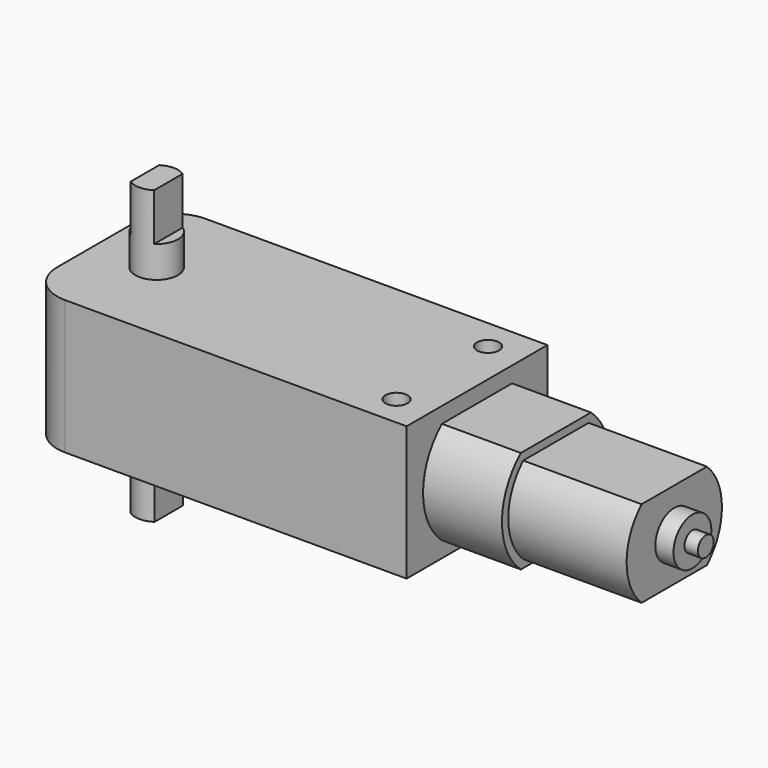
from build123d import *

# Parameters (mm, degrees)
F0_W         = 7.9850807097
F0_H         = 22.3
F0_R         = 1.4
F0_R_2       = 2.7
F1_DEPTH     = 8.5
F0_W_2       = 1.8826620857
F0_H_2       = 1.8826614193
F2_DEPTH     = 1.5
F3_DEPTH     = 18.5
F5_DEPTH     = 10
F6_T         = 1
F6_T3_DEPTH  = 13.109005356
F6_T5_DEPTH  = 5
F6_T7_DEPTH  = 3.8826614193
F6_T10_ANGLE = 98.969647871
F6_T12_ANGLE = 98.969647871
F8_DEPTH     = 15
F9_R         = 3
F9_R_2       = 1.25
F10_DEPTH    = 2.3
F11_DEPTH    = 4
F13_DEPTH    = 6
F15_DEPTH    = 6


# Not quite as in the source:
# - a shell that OpenCascade refuses in one call is made with other operations: the cavity is built on its own and cut out


with BuildPart() as f1:
    # F0 (on Top) → F1 (new body, symmetric)
    with BuildSketch(Plane.XY):
        with Locations((20.1574596452, 0)):
            Rectangle(F0_W, F0_H)
        with Locations((19.75, -7.25)):
            Circle(F0_R, mode=Mode.SUBTRACT)
        with Locations((19.75, 7.25)):
            Circle(F0_R, mode=Mode.SUBTRACT)
        with BuildLine():
            Line((-19.15, -11.15), (16.1649192903, -11.15))
            Line((16.1649192903, -11.15), (16.1649192903, 11.15))
            Line((16.1649192903, 11.15), (-19.15, 11.15))
            ThreePointArc((-19.15, 11.15), (-22.6855339059, 9.6855339059), (-24.15, 6.15))
            Line((-24.15, 6.15), (-24.15, 1.8826614193))
            Line((-24.15, 1.8826614193), (-24.15, 0))
            Line((-24.15, 0), (-24.15, -6.15))
            ThreePointArc((-24.15, -6.15), (-22.6855339059, -9.6855339059), (-19.15, -11.15))
        make_face()
        with Locations((-16.45, 0)):
            Circle(F0_R_2, mode=Mode.SUBTRACT)
    extrude(amount=F1_DEPTH, both=True)

    # F0 (on Top) → F2 (join, symmetric)
    with BuildSketch(Plane.XY):
        with Locations((-25.0913310429, 0.9413307097)):
            Rectangle(F0_W_2, F0_H_2)
    extrude(amount=F2_DEPTH, both=True)

    # F4 (on face) → F5 (join)
    with BuildSketch(Plane.YZ.offset(24.15)):
        with BuildLine():
            Line((5.554502678, 6.5), (-5.554502678, 6.5))
            ThreePointArc((-5.554502678, 6.5), (-8.55, 0), (-5.554502678, -6.5))
            Line((-5.554502678, -6.5), (5.554502678, -6.5))
            ThreePointArc((5.554502678, -6.5), (8.55, 0), (5.554502678, 6.5))
        make_face()
    extrude(amount=F5_DEPTH)

    # F6: shell of thickness 1, made by hand


with BuildPart() as f3:
    # F0 (on Top) → F3 (new body, symmetric)
    with BuildSketch(Plane.XY):
        with Locations((-16.45, 0)):
            Circle(F0_R_2)
    extrude(amount=F3_DEPTH, both=True)

    # F12 (on face) → F13 (cut)
    with BuildSketch(Plane.XY.offset(18.5)):
        with BuildLine():
            ThreePointArc((-17.9390255067, 2.2522884008), (-19.15, 0), (-17.9390255067, -2.2522884008))
            Line((-17.9390255067, -2.2522884008), (-17.9390255067, 2.2522884008))
        make_face()
        with BuildLine():
            Line((-14.9609744933, 2.2522884008), (-14.9609744933, -2.2522884008))
            ThreePointArc((-14.9609744933, -2.2522884008), (-14.0719368314, -1.2785990638), (-13.75, 0))
            ThreePointArc((-13.75, 0), (-14.0719368314, 1.2785990638), (-14.9609744933, 2.2522884008))
        make_face()
    extrude(amount=-F13_DEPTH, mode=Mode.SUBTRACT)

    # F14 (on face) → F15 (cut)
    with BuildSketch(Plane(origin=(0, 0, -18.5), x_dir=(1, 0, 0), z_dir=(0, 0, -1))):
        with BuildLine():
            Line((-17.9761945408, -2.2272696792), (-17.9761945408, 2.2272696792))
            ThreePointArc((-17.9761945408, 2.2272696792), (-19.15, 0), (-17.9761945408, -2.2272696792))
        make_face()
        with BuildLine():
            ThreePointArc((-13.75, 0), (-14.0614099075, 1.2588238042), (-14.9238054592, 2.2272696792))
            Line((-14.9238054592, 2.2272696792), (-14.9238054592, -2.2272696792))
            ThreePointArc((-14.9238054592, -2.2272696792), (-14.0614099075, -1.2588238042), (-13.75, 0))
        make_face()
    extrude(amount=-F15_DEPTH, mode=Mode.SUBTRACT)


with BuildPart() as f6_core1:
    # F6_t2: copy of F1
    add(f1.part)

    # the walls: a layer under each face that stays
    f6_faces = [f6_core1.faces().sort_by_distance(p)[0] for p in [
        (24.15, -7.4333333333, -5.6666666667),
        (0, 0, -8.5),
        (2.5, -11.15, 0),
        (2.5, 11.15, 0),
        (0, 0, 8.5),
        (29.15, 0, -6.5),
        (29.15, 8.55, 0),
        (29.15, 0, 6.5),
        (29.15, -8.55, 0),
        (-22.6855339059, 9.6855339059, 0),
        (-24.15, 4.1, -5.6666666667),
        (-22.6855339059, -9.6855339059, 0),
        (18.35, -7.25, 0),
        (18.35, 7.25, 0),
        (-19.15, 0, 0),
        (-25.0913310429, 1.8826614193, 0),
        (-25.0913310429, 0.9413307097, -1.5),
        (-25.0913310429, 0, 0),
        (-25.0913310429, 0.9413307097, 1.5),
        (-26.0326620857, 0.9413307097, 0),
    ]]
    thicken(f6_faces, amount=-F6_T, mode=Mode.SUBTRACT)

    # F6_s4 → F6_t3 (cut)
    with BuildSketch(Plane.XZ.offset(-6.554502678)):
        Polygon((24.16, -6.51), (23.15, -6.5), (23.15, -5.5), (24.15, -5.5), align=None)
        Polygon((24.16, 6.51), (23.15, 6.5), (23.15, 5.5), (24.15, 5.5), align=None)
    extrude(amount=F6_T3_DEPTH, mode=Mode.SUBTRACT)

    # F6_s6 → F6_t5 (cut)
    with BuildSketch(Plane.XY.offset(-2.5)):
        Polygon((-24.16, 1.8926614193), (-23.15, 1.8826614193), (-23.15, 0.8826614193), (-24.15, 0.8826614193), align=None)
        Polygon((-24.16, -0.01), (-23.15, 0), (-23.15, 1), (-24.15, 1), align=None)
    extrude(amount=F6_T5_DEPTH, mode=Mode.SUBTRACT)

    # F6_s8 → F6_t7 (cut)
    with BuildSketch(Plane.XZ.offset(-2.8826614193)):
        Polygon((-24.16, -1.51), (-23.15, -1.5), (-23.15, -0.5), (-24.15, -0.5), align=None)
        Polygon((-24.16, 1.51), (-23.15, 1.5), (-23.15, 0.5), (-24.15, 0.5), align=None)
    extrude(amount=F6_T7_DEPTH, mode=Mode.SUBTRACT)

    # F6_s9 → F6_t10 (revolve, cut)
    with BuildSketch(Plane(origin=(0, 0, 0), x_dir=(1, 0, 0), z_dir=(0, -0.7602339181, -0.649649436))):
        Polygon((24.16, -8.56), (23.15, -8.55), (23.15, -7.55), (24.15, -7.55), align=None)
    revolve(axis=Axis((24.15, 0, 0), (1, 0, 0)), revolution_arc=F6_T10_ANGLE, mode=Mode.SUBTRACT)

    # F6_s11 → F6_t12 (revolve, cut)
    with BuildSketch(Plane(origin=(0, 0, 0), x_dir=(1, 0, 0), z_dir=(0, 0.7602339181, 0.649649436))):
        Polygon((24.16, -8.56), (23.15, -8.55), (23.15, -7.55), (24.15, -7.55), align=None)
    revolve(axis=Axis((24.15, 0, 0), (1, 0, 0)), revolution_arc=F6_T12_ANGLE, mode=Mode.SUBTRACT)


with BuildPart() as f1_1:
    add(f1.part)

    # what is left inside the walls is the cavity
    f6_cavity = [f6_core1.part.solids().sort_by_distance(p)[0] for p in [
        (0, -3.383333, 7.49),
    ]]
    add(f6_cavity, mode=Mode.SUBTRACT)


with BuildPart() as f8:
    # F7 (on face) → F8 (new body)
    with BuildSketch(Plane.YZ.offset(34.15)):
        with BuildLine():
            Line((5.1722818949, 5.5), (-5.1722818949, 5.5))
            ThreePointArc((-5.1722818949, 5.5), (-7.55, 0), (-5.1722818949, -5.5))
            Line((-5.1722818949, -5.5), (5.1722818949, -5.5))
            ThreePointArc((5.1722818949, -5.5), (7.55, 0), (5.1722818949, 5.5))
        make_face()
    extrude(amount=F8_DEPTH)

    # F9 (on face) → F10 (join)
    with BuildSketch(Plane.YZ.offset(49.15)):
        Circle(F9_R)
        Circle(F9_R_2, mode=Mode.SUBTRACT)
    extrude(amount=F10_DEPTH)

    # F11 (add): a face of the model
    f11_faces = [f8.faces().sort_by_distance(p)[0] for p in [
        (49.15, 0, 0),
    ]]
    extrude(f11_faces, amount=F11_DEPTH)


solid = Compound([f3.part, f1_1.part, f8.part])
